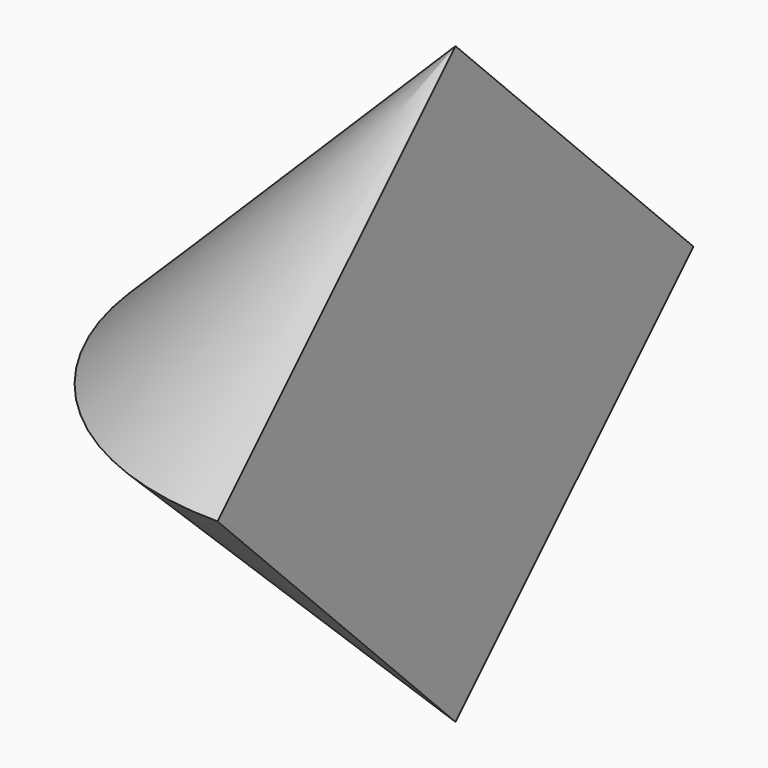
from build123d import *

# Parameters (mm, degrees)
F0_R     = 25
F1_DEPTH = 25
F2_SIZE2 = 24.99999
F2_SIZE  = 24.99999
F3_W     = 55
F3_H     = 55
F4_DEPTH = 30


# Not quite as in the source:
# - a fillet or chamfer is up to 0.001 mm smaller than in the source, because OpenCascade refuses the exact size


with BuildPart() as f1:
    # F0 (on Top) → F1 (new body, symmetric)
    with BuildSketch(Plane.XY):
        Circle(F0_R)
    extrude(amount=F1_DEPTH, both=True)

    # F2 (size 25 and 25 in the source; OpenCascade refuses exactly that, so slightly less here)
    f2_edges = [f1.edges().sort_by_distance(p)[0] for p in [
        (-25, 0, 25),
        (-25, 0, -25),
    ]]
    chamfer(f2_edges, length=F2_SIZE, length2=F2_SIZE2)

    # F3 (on Right) → F4 (cut)
    with BuildSketch(Plane.YZ):
        Rectangle(F3_W, F3_H)
    extrude(amount=F4_DEPTH, mode=Mode.SUBTRACT)


solid = f1.part
